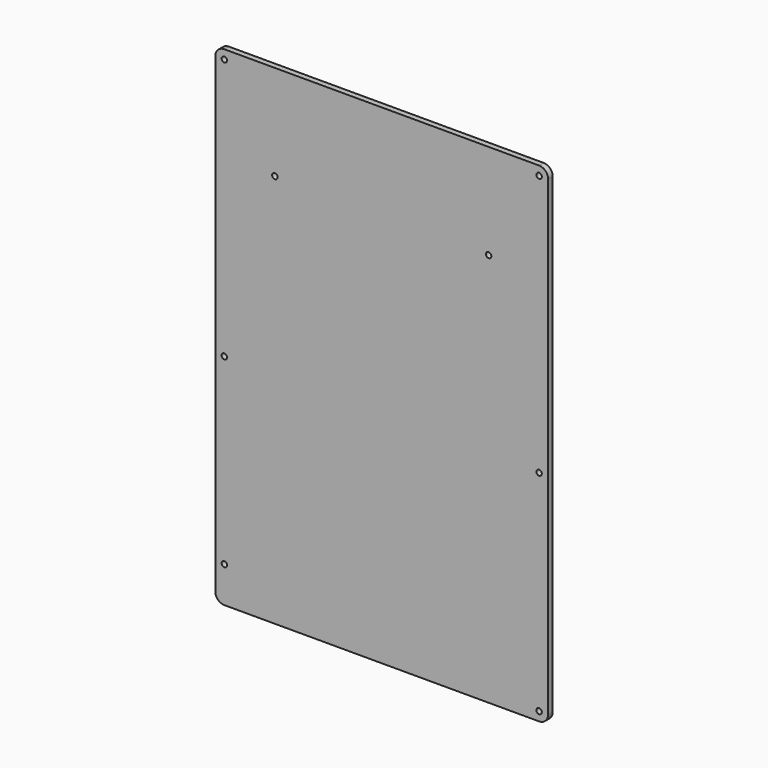
from build123d import *

# Parameters (mm, degrees)
F0_R     = 1.5
F0_W     = 30
F0_H     = 6.7
F0_W_2   = 10
F0_H_2   = 91.46
F0_H_3   = 15
F0_W_3   = 164.6
F0_H_4   = 2.834
F0_H_5   = 5.5
F0_W_4   = 70
F0_H_6   = 1.7
F0_H_7   = 1.48
F0_H_8   = 5
F0_W_5   = 3
F0_H_9   = 1.4
F0_H_10  = 0.6
F1_DEPTH = 3.175


# Not quite as in the source:
# - a feature names something its author has since deleted; it is built from what else it names


with BuildPart() as f1:
    # F0 (on Front) → F1 (new body)
    with BuildSketch(Plane.XZ):
        with BuildLine():
            Line((-18.7680281997, 132.5136111658), (-91.7680281997, 132.5136111658))
            ThreePointArc((-91.7680281997, 132.5136111658), (-95.3035621056, 131.0491450717), (-96.7680281997, 127.5136111658))
            Line((-96.7680281997, 127.5136111658), (-96.7680281997, -22.4863888342))
            Line((-96.7680281997, -22.4863888342), (-86.7680281997, -22.4863888342))
            Line((-86.7680281997, -22.4863888342), (-86.7680281997, 13.1196111658))
            Line((-86.7680281997, 13.1196111658), (-86.7680281997, 15.9536111658))
            Line((-86.7680281997, 15.9536111658), (-86.7680281997, 21.4536111658))
            Line((-86.7680281997, 21.4536111658), (-89.7680281997, 21.4536111658))
            Line((-89.7680281997, 21.4536111658), (-89.7680281997, 22.0536111658))
            Line((-89.7680281997, 22.0536111658), (-89.7680281997, 22.8536111658))
            Line((-89.7680281997, 22.8536111658), (-89.7680281997, 23.4536111658))
            Line((-89.7680281997, 23.4536111658), (-86.7680281997, 23.4536111658))
            Line((-86.7680281997, 23.4536111658), (-86.7680281997, 24.6436111658))
            Line((-86.7680281997, 24.6436111658), (-86.7680281997, 53.4536111658))
            Line((-86.7680281997, 53.4536111658), (-86.7680281997, 60.9536111658))
            Line((-86.7680281997, 60.9536111658), (-86.7680281997, 64.0936111658))
            Line((-86.7680281997, 64.0936111658), (-86.7680281997, 122.5136111658))
            Line((-86.7680281997, 122.5136111658), (-40.4680281997, 122.5136111658))
            Line((-40.4680281997, 122.5136111658), (-39.4680281997, 122.5136111658))
            Line((-39.4680281997, 122.5136111658), (-39.4680281997, 124.2136111658))
            Line((-39.4680281997, 124.2136111658), (-49.4680281997, 124.2136111658))
            Line((-49.4680281997, 124.2136111658), (-49.4680281997, 125.8136111658))
            Line((-49.4680281997, 125.8136111658), (-28.7680281997, 125.8136111658))
            Line((-28.7680281997, 125.8136111658), (-18.7680281997, 125.8136111658))
            Line((-18.7680281997, 125.8136111658), (-18.7680281997, 132.5136111658))
        make_face()
        with Locations((-91.7680281997, -17.4863888342)):
            Circle(F0_R, mode=Mode.SUBTRACT)
        with Locations((-91.7680281997, 127.5136111658)):
            Circle(F0_R, mode=Mode.SUBTRACT)
        with Locations((-3.7680281997, 129.1636111658)):
            Rectangle(F0_W, F0_H)
        with BuildLine():
            Line((82.8319718003, 132.5136111658), (11.2319718003, 132.5136111658))
            Line((11.2319718003, 132.5136111658), (11.2319718003, 125.8136111658))
            Line((11.2319718003, 125.8136111658), (21.2319718003, 125.8136111658))
            Line((21.2319718003, 125.8136111658), (40.5319718003, 125.8136111658))
            Line((40.5319718003, 125.8136111658), (40.5319718003, 124.2136111658))
            Line((40.5319718003, 124.2136111658), (30.5319718003, 124.2136111658))
            Line((30.5319718003, 124.2136111658), (30.5319718003, 122.5136111658))
            Line((30.5319718003, 122.5136111658), (40.5319718003, 122.5136111658))
            Line((40.5319718003, 122.5136111658), (77.8319718003, 122.5136111658))
            Line((77.8319718003, 122.5136111658), (77.8319718003, 64.0936111658))
            Line((77.8319718003, 64.0936111658), (77.8319718003, 60.9536111658))
            Line((77.8319718003, 60.9536111658), (77.8319718003, 53.4536111658))
            Line((77.8319718003, 53.4536111658), (77.8319718003, 24.6436111658))
            Line((77.8319718003, 24.6436111658), (77.8319718003, 23.4536111658))
            Line((77.8319718003, 23.4536111658), (80.8319718003, 23.4536111658))
            Line((80.8319718003, 23.4536111658), (80.8319718003, 22.8536111658))
            Line((80.8319718003, 22.8536111658), (80.8319718003, 21.4536111658))
            Line((80.8319718003, 21.4536111658), (77.8319718003, 21.4536111658))
            Line((77.8319718003, 21.4536111658), (77.8319718003, 15.9536111658))
            Line((77.8319718003, 15.9536111658), (77.8319718003, 13.1196111658))
            Line((77.8319718003, 13.1196111658), (77.8319718003, -128.9463888342))
            Line((77.8319718003, -128.9463888342), (1.2319718003, -128.9463888342))
            Line((1.2319718003, -128.9463888342), (1.2319718003, -130.4263888342))
            Line((1.2319718003, -130.4263888342), (3.7319718003, -130.4263888342))
            Line((3.7319718003, -130.4263888342), (3.7319718003, -132.0263888342))
            Line((3.7319718003, -132.0263888342), (-11.2680281997, -132.0263888342))
            Line((-11.2680281997, -132.0263888342), (-11.2680281997, -130.4263888342))
            Line((-11.2680281997, -130.4263888342), (-8.7680281997, -130.4263888342))
            Line((-8.7680281997, -130.4263888342), (-8.7680281997, -128.9463888342))
            Line((-8.7680281997, -128.9463888342), (-86.7680281997, -128.9463888342))
            Line((-86.7680281997, -128.9463888342), (-96.7680281997, -128.9463888342))
            Line((-96.7680281997, -128.9463888342), (-96.7680281997, -132.2803888342))
            Line((-96.7680281997, -132.2803888342), (-96.7680281997, -133.9463888342))
            ThreePointArc((-96.7680281997, -133.9463888342), (-95.3035621056, -137.4819227401), (-91.7680281997, -138.9463888342))
            Line((-91.7680281997, -138.9463888342), (82.8319718003, -138.9463888342))
            ThreePointArc((82.8319718003, -138.9463888342), (86.3675057063, -137.4819227401), (87.8319718003, -133.9463888342))
            Line((87.8319718003, -133.9463888342), (87.8319718003, 127.5136111658))
            ThreePointArc((87.8319718003, 127.5136111658), (86.3675057063, 131.0491450717), (82.8319718003, 132.5136111658))
        make_face()
        with Locations((82.8319718003, -133.9463888342)):
            Circle(F0_R, mode=Mode.SUBTRACT)
        with Locations((82.8319718003, -17.4863888342)):
            Circle(F0_R, mode=Mode.SUBTRACT)
        with Locations((82.8319718003, 127.5136111658)):
            Circle(F0_R, mode=Mode.SUBTRACT)
        Polygon((11.2319718003, 125.8136111658), (-18.7680281997, 125.8136111658), (-28.7680281997, 125.8136111658), (-49.4680281997, 125.8136111658), (-49.4680281997, 124.2136111658), (-39.4680281997, 124.2136111658), (30.5319718003, 124.2136111658), (40.5319718003, 124.2136111658), (40.5319718003, 125.8136111658), (21.2319718003, 125.8136111658), align=None)
        with Locations((-91.7680281997, -68.2163888342)):
            Rectangle(F0_W_2, F0_H_2)
        with Locations((-91.7680281997, -121.4463888342)):
            Rectangle(F0_W_2, F0_H_3)
        with Locations((-91.7680281997, -118.9463888342)):
            Circle(F0_R, mode=Mode.SUBTRACT)
        Polygon((-86.7680281997, 13.1196111658), (-86.7680281997, -22.4863888342), (-86.7680281997, -113.9463888342), (-86.7680281997, -128.9463888342), (-8.7680281997, -128.9463888342), (1.2319718003, -128.9463888342), (77.8319718003, -128.9463888342), (77.8319718003, 13.1196111658), align=None)
        with Locations((-4.4680281997, 14.5366111658)):
            Rectangle(F0_W_3, F0_H_4)
        with Locations((-4.4680281997, 18.7036111658)):
            Rectangle(F0_W_3, F0_H_5)
        with Locations((-4.4680281997, 123.3636111658)):
            Rectangle(F0_W_4, F0_H_6)
        with Locations((-3.7680281997, -129.6863888342)):
            Rectangle(F0_W_2, F0_H_7)
        Polygon((-89.7680281997, 21.4536111658), (-86.7680281997, 21.4536111658), (-86.7680281997, 22.0536111658), (-86.7680281997, 22.8536111658), (-89.7680281997, 22.8536111658), (-89.7680281997, 22.0536111658), align=None)
        Polygon((-86.7680281997, 22.0536111658), (-86.7680281997, 21.4536111658), (77.8319718003, 21.4536111658), (77.8319718003, 22.8536111658), (77.8319718003, 23.4536111658), (-86.7680281997, 23.4536111658), (-86.7680281997, 22.8536111658), align=None)
        Polygon((-39.4680281997, 117.5136111658), (-39.4680281997, 122.5136111658), (-40.4680281997, 122.5136111658), (-86.7680281997, 122.5136111658), (-86.7680281997, 64.0936111658), (-66.675587153, 64.0936111658), align=None)
        with Locations((-63.7680281997, 79.6436111658)):
            Circle(F0_R, mode=Mode.SUBTRACT)
        with Locations((-4.4680281997, 120.0136111658)):
            Rectangle(F0_W_4, F0_H_8)
        Polygon((1.2319718003, -130.4263888342), (-8.7680281997, -130.4263888342), (-11.2680281997, -130.4263888342), (-11.2680281997, -132.0263888342), (3.7319718003, -132.0263888342), (3.7319718003, -130.4263888342), align=None)
        with Locations((79.3319718003, 22.1536111658)):
            Rectangle(F0_W_5, F0_H_9)
        Polygon((40.5319718003, 122.5136111658), (30.5319718003, 122.5136111658), (30.5319718003, 117.5136111658), (57.7395307537, 64.0936111658), (77.8319718003, 64.0936111658), (77.8319718003, 122.5136111658), align=None)
        with Locations((54.8319718003, 79.6436111658)):
            Circle(F0_R, mode=Mode.SUBTRACT)
        Polygon((30.5319718003, 117.5136111658), (-39.4680281997, 117.5136111658), (-66.675587153, 64.0936111658), (57.7395307537, 64.0936111658), align=None)
        with Locations((-88.2680281997, 23.1536111658)):
            Rectangle(F0_W_5, F0_H_10)
        with Locations((79.3319718003, 23.1536111658)):
            Rectangle(F0_W_5, F0_H_10)
        Polygon((57.7395307537, 64.0936111658), (-66.675587153, 64.0936111658), (-68.2748334113, 60.9536111658), (59.3387770119, 60.9536111658), align=None)
        Polygon((-68.2748334113, 60.9536111658), (-66.675587153, 64.0936111658), (-86.7680281997, 64.0936111658), (-86.7680281997, 60.9536111658), align=None)
        Polygon((-86.7680281997, 24.6436111658), (-86.7680281997, 23.4536111658), (77.8319718003, 23.4536111658), (77.8319718003, 24.6436111658), (63.1586327242, 53.4536111658), (-72.0946891235, 53.4536111658), align=None)
        Polygon((77.8319718003, 64.0936111658), (57.7395307537, 64.0936111658), (59.3387770119, 60.9536111658), (77.8319718003, 60.9536111658), align=None)
        Polygon((59.3387770119, 60.9536111658), (-68.2748334113, 60.9536111658), (-72.0946891235, 53.4536111658), (63.1586327242, 53.4536111658), align=None)
        Polygon((-72.0946891235, 53.4536111658), (-68.2748334113, 60.9536111658), (-86.7680281997, 60.9536111658), (-86.7680281997, 53.4536111658), align=None)
        Polygon((-86.7680281997, 53.4536111658), (-86.7680281997, 24.6436111658), (-72.0946891235, 53.4536111658), align=None)
        Polygon((63.1586327242, 53.4536111658), (77.8319718003, 24.6436111658), (77.8319718003, 53.4536111658), align=None)
        Polygon((77.8319718003, 60.9536111658), (59.3387770119, 60.9536111658), (63.1586327242, 53.4536111658), (77.8319718003, 53.4536111658), align=None)
    extrude(amount=F1_DEPTH)


solid = f1.part
